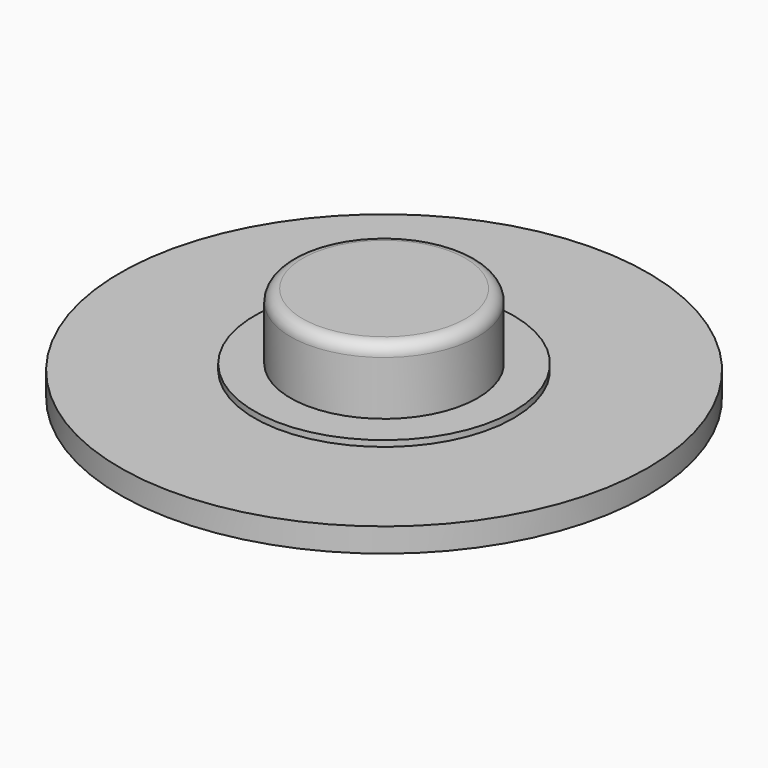
from build123d import *

# Parameters (mm, degrees)
F2_R     = 11
F2_R_2   = 5.4
F2_R_3   = 3.9
F3_DEPTH = 1
F4_DEPTH = 3
F5_DEPTH = 0.25
F6_R     = 0.5


# Not quite as in the source:
# - a feature names something its author has since deleted; it is built from what else it names


with BuildPart() as f3:
    # F2 (on Top) → F3 (new body)
    with BuildSketch(Plane.XY):
        Circle(F2_R)
        Circle(F2_R_2, mode=Mode.SUBTRACT)
        Circle(F2_R_2)
        Circle(F2_R_3, mode=Mode.SUBTRACT)
        Circle(F2_R_3)
    extrude(amount=-F3_DEPTH)

    # F2 (on Top) → F4 (join)
    with BuildSketch(Plane.XY):
        Circle(F2_R_3)
    extrude(amount=F4_DEPTH)

    # F2 (on Top) → F5 (join)
    with BuildSketch(Plane.XY):
        Circle(F2_R_2)
        Circle(F2_R_3, mode=Mode.SUBTRACT)
    extrude(amount=F5_DEPTH)

    # F6
    f6_edges = [f3.edges().sort_by_distance(p)[0] for p in [
        (-3.9, 0, 3),
    ]]
    fillet(f6_edges, radius=F6_R)


solid = f3.part
